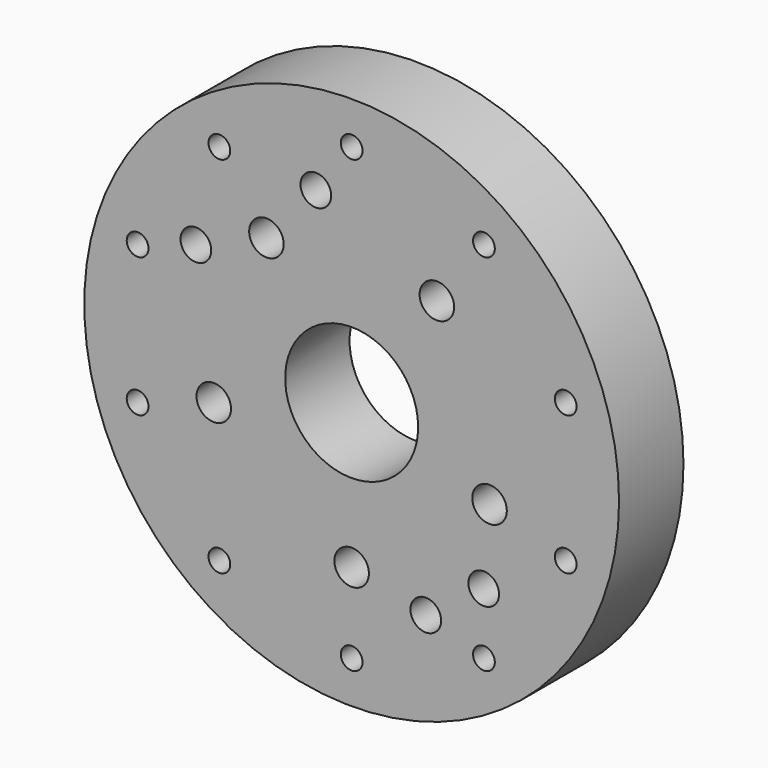
from build123d import *

# Parameters (mm, degrees)
F0_R     = 82.9945
F0_R_2   = 7.9375
F0_R_3   = 20.6375
F0_R_4   = 4.7625
F1_DEPTH = 25
F2_D     = 6.7564
F3_DEPTH = 6.35
F5_D     = 10.71626


# Not quite as in the source:
# - a feature names something its author has since deleted; it is built from what else it names


with BuildPart() as f1:
    # F0 (on Front) → F1 (new body)
    with BuildSketch(Plane.XZ):
        Circle(F0_R)
        with Locations((-23.0087746099, -50.5745756008)):
            Circle(F0_R_2, mode=Mode.SUBTRACT)
        with Locations((-40.9891773098, -37.5110483686)):
            Circle(F0_R_2, mode=Mode.SUBTRACT)
        with Locations((23.0087746099, -50.5745756008)):
            Circle(F0_R_2, mode=Mode.SUBTRACT)
        with Locations((40.9891773098, -37.5110483686)):
            Circle(F0_R_2, mode=Mode.SUBTRACT)
        with Locations((-55.2093820582, 6.2542416807)):
            Circle(F0_R_2, mode=Mode.SUBTRACT)
        with Locations((-48.3414793582, 27.3914727554)):
            Circle(F0_R_2, mode=Mode.SUBTRACT)
        with Locations((-11.1125, 54.4399095334)):
            Circle(F0_R_2, mode=Mode.SUBTRACT)
        Circle(F0_R_3, mode=Mode.SUBTRACT)
        with Locations((55.2093820582, 6.2542416807)):
            Circle(F0_R_2, mode=Mode.SUBTRACT)
        with Locations((48.3414793582, 27.3914727554)):
            Circle(F0_R_2, mode=Mode.SUBTRACT)
        with Locations((11.1125, 54.4399095334)):
            Circle(F0_R_2, mode=Mode.SUBTRACT)
        with Locations((-48.3414793582, 27.3914727554)):
            Circle(F0_R_2)
        with Locations((-48.3414793582, 27.3914727554)):
            Circle(F0_R_4, mode=Mode.SUBTRACT)
        with Locations((-11.1125, 54.4399095334)):
            Circle(F0_R_2)
        with Locations((-11.1125, 54.4399095334)):
            Circle(F0_R_4, mode=Mode.SUBTRACT)
        with Locations((-55.2093820582, 6.2542416807)):
            Circle(F0_R_2)
        with Locations((-55.2093820582, 6.2542416807)):
            Circle(F0_R_4, mode=Mode.SUBTRACT)
        with Locations((-40.9891773098, -37.5110483686)):
            Circle(F0_R_2)
        with Locations((-40.9891773098, -37.5110483686)):
            Circle(F0_R_4, mode=Mode.SUBTRACT)
        with Locations((-23.0087746099, -50.5745756008)):
            Circle(F0_R_2)
        with Locations((-23.0087746099, -50.5745756008)):
            Circle(F0_R_4, mode=Mode.SUBTRACT)
        with Locations((55.2093820582, 6.2542416807)):
            Circle(F0_R_2)
        with Locations((55.2093820582, 6.2542416807)):
            Circle(F0_R_4, mode=Mode.SUBTRACT)
        with Locations((48.3414793582, 27.3914727554)):
            Circle(F0_R_2)
        with Locations((48.3414793582, 27.3914727554)):
            Circle(F0_R_4, mode=Mode.SUBTRACT)
        with Locations((11.1125, 54.4399095334)):
            Circle(F0_R_2)
        with Locations((11.1125, 54.4399095334)):
            Circle(F0_R_4, mode=Mode.SUBTRACT)
        with Locations((23.0087746099, -50.5745756008)):
            Circle(F0_R_2)
        with Locations((23.0087746099, -50.5745756008)):
            Circle(F0_R_4, mode=Mode.SUBTRACT)
        with Locations((40.9891773098, -37.5110483686)):
            Circle(F0_R_2)
        with Locations((40.9891773098, -37.5110483686)):
            Circle(F0_R_4, mode=Mode.SUBTRACT)
        with Locations((-55.2093820582, 6.2542416807)):
            Circle(F0_R_4)
        with Locations((-40.9891773098, -37.5110483686)):
            Circle(F0_R_4)
        with Locations((-23.0087746099, -50.5745756008)):
            Circle(F0_R_4)
        with Locations((55.2093820582, 6.2542416807)):
            Circle(F0_R_4)
        with Locations((48.3414793582, 27.3914727554)):
            Circle(F0_R_4)
        with Locations((11.1125, 54.4399095334)):
            Circle(F0_R_4)
    extrude(amount=F1_DEPTH)

    # F2 (through all)
    with Locations(Plane(origin=(0, 0, 0), x_dir=(1, 0, 0), z_dir=(0, 1, 0))):
        with Locations((0, -69.85), (41.0567998726, -56.5098370571), (66.4312976632, -21.5848370571), (66.4312976632, 21.5848370571), (41.0567998726, 56.5098370571), (0, 69.85), (-41.0567998726, 56.5098370571), (-66.4312976632, 21.5848370571), (-66.4312976632, -21.5848370571), (-41.0567998726, -56.5098370571)):
            Hole(F2_D / 2)

    # F0 (on Front) → F3 (cut)
    with BuildSketch(Plane.XZ):
        with Locations((-11.1125, 54.4399095334)):
            Circle(F0_R_2)
        with Locations((-11.1125, 54.4399095334)):
            Circle(F0_R_4, mode=Mode.SUBTRACT)
        with Locations((-48.3414793582, 27.3914727554)):
            Circle(F0_R_2)
        with Locations((-48.3414793582, 27.3914727554)):
            Circle(F0_R_4, mode=Mode.SUBTRACT)
        with Locations((40.9891773098, -37.5110483686)):
            Circle(F0_R_2)
        with Locations((40.9891773098, -37.5110483686)):
            Circle(F0_R_4, mode=Mode.SUBTRACT)
        with Locations((23.0087746099, -50.5745756008)):
            Circle(F0_R_2)
        with Locations((23.0087746099, -50.5745756008)):
            Circle(F0_R_4, mode=Mode.SUBTRACT)
    extrude(amount=F3_DEPTH, mode=Mode.SUBTRACT)

    # F5 (through all)
    with Locations(Plane(origin=(0, 0, 0), x_dir=(1, 0, 0), z_dir=(0, 1, 0))):
        with Locations((0, 45), (42.7975432333, 13.9057647469), (26.4503363532, -36.4057647469), (-26.4503363532, -36.4057647469), (-42.7975432333, 13.9057647469)):
            Hole(F5_D / 2)


solid = f1.part
